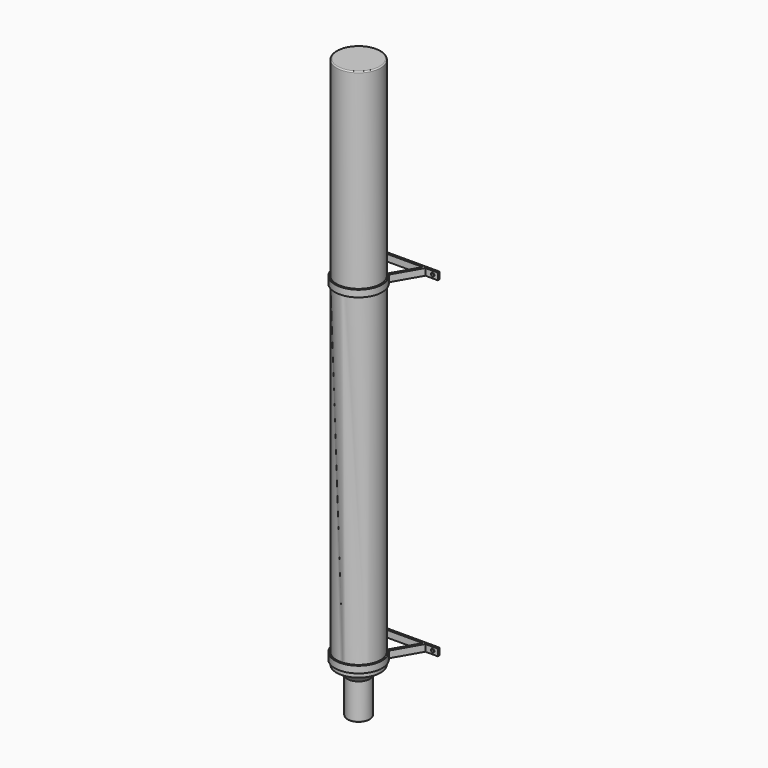
from build123d import *

# Parameters (mm, degrees)
F0_R      = 98
F1_DEPTH  = 1284.5
F2_R      = 98
F2_R_2    = 50
F3_DEPTH  = 200
F4_SIZE   = 40
F5_R      = 5
F8_DEPTH  = 30
F9_R      = 6.75
F9_R_2    = 7.5
F10_DEPTH = 10.001


# Not quite as in the source:
# - a pattern or mirror of a feature is missing from the dataset's text; its kind, count and spacing are read off the source's solid


with BuildPart() as f1:
    # F0 (on Top) → F1 (new body, symmetric)
    with BuildSketch(Plane.XY):
        Circle(F0_R)
    extrude(amount=F1_DEPTH, both=True)

    # F2 (on face) → F3 (cut)
    with BuildSketch(Plane(origin=(0, 0, -1284.5), x_dir=(1, 0, 0), z_dir=(0, 0, -1))):
        Circle(F2_R)
        Circle(F2_R_2, mode=Mode.SUBTRACT)
    extrude(amount=-F3_DEPTH, mode=Mode.SUBTRACT)

    # F4
    f4_edges = [f1.edges().sort_by_distance(p)[0] for p in [
        (-50, 0, -1084.5),
    ]]
    chamfer(f4_edges, length=F4_SIZE)

    # F5
    f5_edges = [f1.edges().sort_by_distance(p)[0] for p in [
        (-50, 0, -1284.5),
        (-98, 0, 1284.5),
    ]]
    fillet(f5_edges, radius=F5_R)

    # F7 (on offset) → F8 (join)
    with BuildSketch(Plane(origin=(0, 0, -1064.5), x_dir=(1, 0, 0), z_dir=(0, 0, -1))):
        Polygon((76.2233031652, -72.2150126676), (65.2159465136, -73.14971169), (132.6794919243, -190), (-132.6794919243, -190), (-65.2159465136, -73.14971169), (-76.2233031652, -72.2150126676), (-144.2264973081, -190), (-200, -190), (-200, -200), (-150, -200), (150, -200), (200, -200), (200, -190), (144.2264973081, -190), align=None)
        with BuildLine():
            ThreePointArc((-65.2159465136, -73.14971169), (0, 98), (65.2159465136, -73.14971169))
            Line((65.2159465136, -73.14971169), (76.2233031652, -72.2150126676))
            ThreePointArc((76.2233031652, -72.2150126676), (0, 105), (-76.2233031652, -72.2150126676))
            Line((-76.2233031652, -72.2150126676), (-65.2159465136, -73.14971169))
        make_face()
    f8 = extrude(amount=-F8_DEPTH)

    # F8_copies: F8 across plane
    add(f8.mirror(Plane.XY.offset(-314.5)))

    # F9 (on face) → F10 (cut, through all)
    with BuildSketch(Plane.XZ.offset(-190)):
        with Locations((-172.1132486541, -1049.5)):
            Circle(F9_R)
        with Locations((176.858574152, -1049.5)):
            Circle(F9_R_2)
    f10 = extrude(amount=-F10_DEPTH, mode=Mode.SUBTRACT)

    # F10_copies: F10 across plane
    add(f10.mirror(Plane.XY.offset(-314.5)), mode=Mode.SUBTRACT)


solid = f1.part
